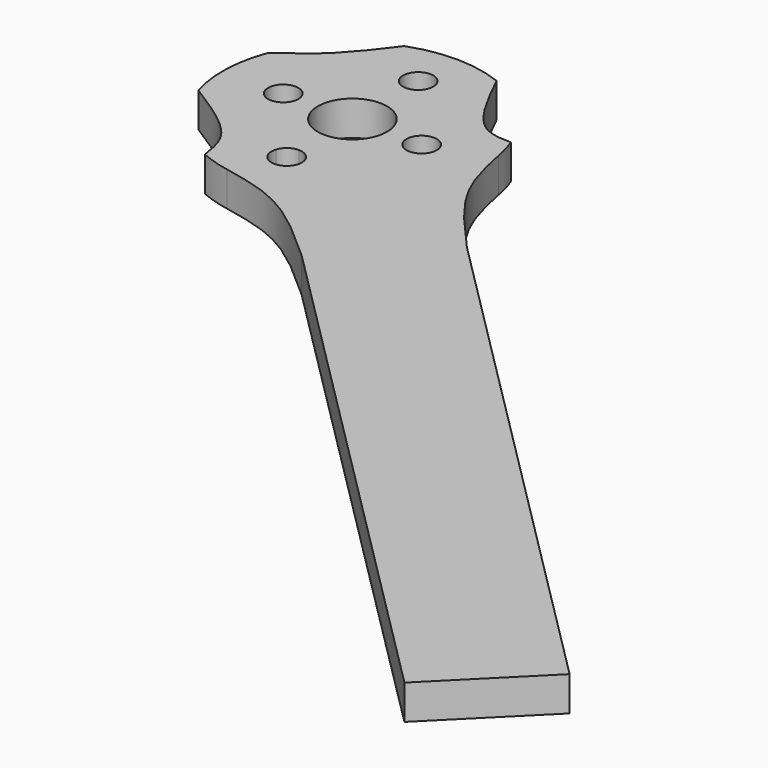
from build123d import *

# Parameters (mm, degrees)
F0_R     = 1.75
F1_DEPTH = 4


with BuildPart() as f1:
    # F0 (on Top) → F1 (new body)
    with BuildSketch(Plane.XY):
        with BuildLine():
            Line((6.0892546755, -33.3552707336), (11.3925555344, -28.0519698747))
            Line((11.3925555344, -28.0519698747), (-9.3547162967, -7.3046980436))
            Line((-9.3547162967, -7.3046980436), (-55.7825886783, 39.1231743381))
            ThreePointArc((-55.7825886783, 39.1231743381), (-58.8891903961, 36.7393949991), (-62.5069047196, 35.2408886615))
            Line((-62.5069047196, 35.2408886615), (-53.2885795254, 26.0225634673))
            Line((-53.2885795254, 26.0225634673), (6.0892546755, -33.3552707336))
        make_face()
        with BuildLine():
            Line((-9.3547162967, -7.3046980436), (11.3925555344, -28.0519698747))
            Line((11.3925555344, -28.0519698747), (16.6958563933, -22.7486690158))
            Line((16.6958563933, -22.7486690158), (-42.6819778076, 36.6291651851))
            add(Edge.make_bspline(
                [(-42.6819778076, 36.6291651851), (-45.2945511903, 39.5061130095), (-50.0695074398, 44.7616576166), (-51.1430333829, 50.0297724966), (-51.6312848813, 52.4138447612)],
                knots=[0, 0, 0, 0, 0.5473526332, 1, 1, 1, 1], degree=3))
            ThreePointArc((-51.6312848813, 52.4138447612), (-51.4017631208, 49.1157535279), (-51.9003030018, 45.8474903793))
            ThreePointArc((-51.9003030018, 45.8474903793), (-53.3988093394, 42.2297760559), (-55.7825886783, 39.1231743381))
            Line((-55.7825886783, 39.1231743381), (-9.3547162967, -7.3046980436))
        make_face()
        with BuildLine():
            ThreePointArc((-62.5069047196, 35.2408886615), (-58.8891903961, 36.7393949991), (-55.7825886783, 39.1231743381))
            ThreePointArc((-55.7825886783, 39.1231743381), (-53.3988093394, 42.2297760559), (-51.9003030018, 45.8474903793))
            ThreePointArc((-51.9003030018, 45.8474903793), (-51.4017631208, 49.1157535279), (-51.6312848813, 52.4138447612))
            ThreePointArc((-51.6312848813, 52.4138447612), (-51.9458010107, 53.7780476698), (-52.3861331822, 55.1069861748))
            add(Edge.make_bspline(
                [(-52.3861331822, 55.1069861748), (-53.6051347333, 55.1308330266), (-56.7515994276, 55.1918775104), (-59.3237157089, 60.4625666695), (-60.9000344454, 63.6893307389)],
                knots=[0, 0, 0, 0, 0.387493123, 1, 1, 1, 1], degree=3))
            ThreePointArc((-60.9000344454, 63.6893307389), (-66.2678346698, 64.7292851408), (-71.6517589086, 63.7763191413))
            add(Edge.make_bspline(
                [(-80.3976496024, 55.0928974107), (-78.8782096295, 56.1643689504), (-75.6891919016, 58.3945745707), (-73.0396610336, 61.9384087083), (-71.6517589086, 63.7763191413)],
                knots=[0, 0, 0, 0, 0.4784709271, 1, 1, 1, 1], degree=3))
            ThreePointArc((-80.3976496024, 55.0928974107), (-81.3784942248, 50.296142309), (-80.7624173443, 45.4390480176))
            add(Edge.make_bspline(
                [(-72.4758721042, 36.0202061945), (-72.6700492153, 37.3502311658), (-73.1313035357, 40.642383964), (-77.9288722558, 43.6485061475), (-80.7624173443, 45.4390480176)],
                knots=[0, 0, 0, 0, 0.4064160365, 1, 1, 1, 1], degree=3))
            ThreePointArc((-72.4758721042, 36.0202061945), (-70.8057804399, 35.3947234788), (-69.0732591015, 34.971870541))
            ThreePointArc((-69.0732591015, 34.971870541), (-65.7751678682, 34.7423487805), (-62.5069047196, 35.2408886615))
        make_face()
        with Locations((-74.3891903961, 49.7297760559)):
            Circle(F0_R, mode=Mode.SUBTRACT)
        with BuildLine():
            ThreePointArc((-64.6391903961, 40.2297760559), (-64.9694713976, 39.2065957368), (-65.8356452136, 38.5696291555))
            ThreePointArc((-65.8356452136, 38.5696291555), (-67.6266272632, 38.9923391888), (-68.0493372965, 40.7833212384))
            ThreePointArc((-68.0493372965, 40.7833212384), (-67.4123707152, 41.6494950544), (-66.3891903961, 41.9797760559))
            ThreePointArc((-66.3891903961, 41.9797760559), (-65.1517535291, 41.4672129229), (-64.6391903961, 40.2297760559))
        make_face(mode=Mode.SUBTRACT)
        with BuildLine():
            ThreePointArc((-62.3891903961, 49.7297760559), (-62.6936722661, 48.1990423264), (-63.5607632714, 46.9013489311))
            ThreePointArc((-63.5607632714, 46.9013489311), (-70.0847085262, 51.2605097853), (-62.3891903961, 49.7297760559))
        make_face(mode=Mode.SUBTRACT)
        with BuildLine():
            ThreePointArc((-60.1391903961, 49.7297760559), (-58.3891903961, 51.4797760559), (-56.6391903961, 49.7297760559))
            ThreePointArc((-56.6391903961, 49.7297760559), (-58.3891903961, 47.9797760559), (-60.1391903961, 49.7297760559))
        make_face(mode=Mode.SUBTRACT)
        with BuildLine():
            ThreePointArc((-66.3891903961, 57.4797760559), (-67.6266272632, 60.4672129229), (-64.6391903961, 59.2297760559))
            ThreePointArc((-64.6391903961, 59.2297760559), (-65.1517535291, 57.9923391888), (-66.3891903961, 57.4797760559))
        make_face(mode=Mode.SUBTRACT)
        with BuildLine():
            add(Edge.make_bspline(
                [(-53.2885795254, 26.0225634673), (-56.1655273498, 28.63513685), (-61.4210719568, 33.4100930995), (-66.6891868368, 34.4836190426), (-69.0732591015, 34.971870541)],
                knots=[0, 0, 0, 0, 0.5473526332, 1, 1, 1, 1], degree=3))
            Line((-53.2885795254, 26.0225634673), (-62.5069047196, 35.2408886615))
            ThreePointArc((-62.5069047196, 35.2408886615), (-65.7751678682, 34.7423487805), (-69.0732591015, 34.971870541))
        make_face()
    extrude(amount=F1_DEPTH)


solid = f1.part
